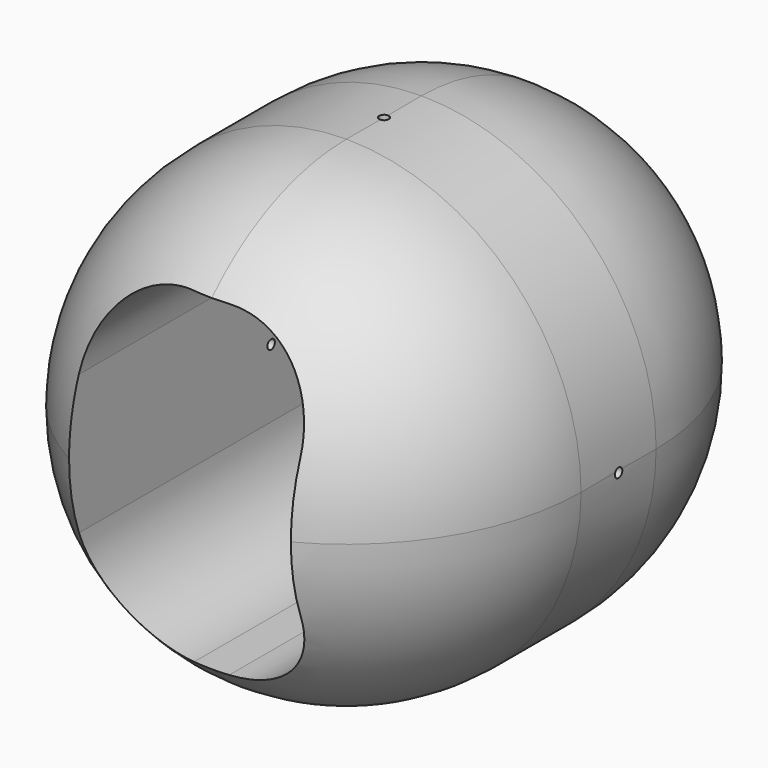
from build123d import *

# Parameters (mm, degrees)
F0_W          = 127
F0_H          = 127
F1_DEPTH      = 152.4
F2_R          = 63.49999
F3_W          = 60.3535668924
F3_H          = 88.5923877358
F4_DEPTH      = 187.706
F5_R          = 25.4
F6_R          = 1.27
F7_DEPTH      = 62.9846544394
F7_DEPTH_BACK = 95.758
F8_R          = 1.27
F9_DEPTH      = 78.9673156079
F9_DEPTH_BACK = 48.0346845921


# Not quite as in the source:
# - a fillet or chamfer is up to 0.001 mm smaller than in the source, because OpenCascade refuses the exact size


with BuildPart() as f1:
    # F0 (on Front) → F1 (new body)
    with BuildSketch(Plane.XZ):
        with Locations((15.4663155079, 0.5163455606)):
            Rectangle(F0_W, F0_H)
    extrude(amount=F1_DEPTH)

    # F2 (radius 63.5 in the source; OpenCascade refuses exactly that, so slightly less here)
    f2_edges = [f1.edges().sort_by_distance(p)[0] for p in [
        (-48.033684, -76.2, 64.016346),
        (-48.033684, -152.4, 0.516346),
        (15.466316, -152.4, 64.016346),
        (78.966316, -152.4, 0.516346),
        (78.966316, -76.2, 64.016346),
        (78.966316, 0, 0.516346),
        (15.466316, 0, -62.983654),
        (78.966316, -76.2, -62.983654),
        (-48.033684, -76.2, -62.983654),
        (-48.033684, 0, 0.516346),
        (15.466316, -152.4, -62.983654),
        (15.466316, 0, 64.016346),
    ]]
    fillet(f2_edges, radius=F2_R)

    # F3 (on Front) → F4 (cut)
    with BuildSketch(Plane.XZ):
        with Locations((15.0872929953, 0.415276736)):
            Rectangle(F3_W, F3_H)
    extrude(amount=F4_DEPTH, mode=Mode.SUBTRACT)

    # F5
    f5_edges = [f1.edges().sort_by_distance(p)[0] for p in [
        (45.264076, -76.2, -43.880917),
        (45.264076, -76.2, 44.711471),
        (-15.08949, -76.2, 44.711471),
        (-15.08949, -76.2, -43.880917),
    ]]
    fillet(f5_edges, radius=F5_R)

    # F6 (on Top) → F7 (cut, two sides)
    with BuildSketch(Plane.XY) as f7_sk:
        with Locations((15.4663155079, -76.2)):
            Circle(F6_R)
    extrude(amount=-F7_DEPTH, mode=Mode.SUBTRACT)
    extrude(f7_sk.sketch, amount=F7_DEPTH_BACK, mode=Mode.SUBTRACT)

    # F8 (on Right) → F9 (cut, two sides)
    with BuildSketch(Plane.YZ) as f9_sk:
        with Locations((-76.2, 0)):
            Circle(F8_R)
    extrude(amount=F9_DEPTH, mode=Mode.SUBTRACT)
    extrude(f9_sk.sketch, amount=-F9_DEPTH_BACK, mode=Mode.SUBTRACT)


solid = f1.part
